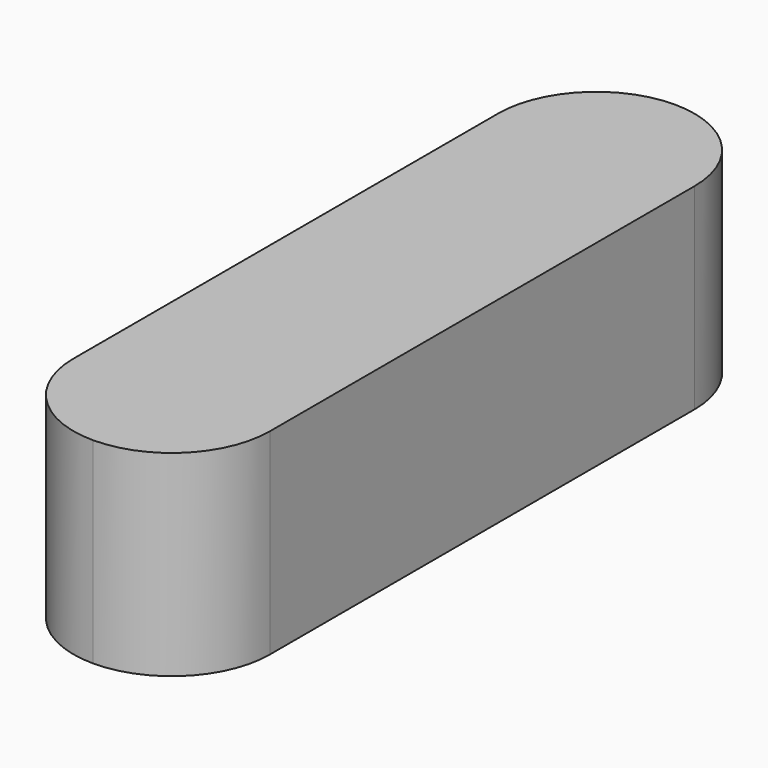
from build123d import *

# Parameters (mm, degrees)
F0_W     = 10
F0_H     = 37
F1_DEPTH = 10
F2_R     = 4.99999


# Not quite as in the source:
# - a fillet or chamfer is up to 0.001 mm smaller than in the source, because OpenCascade refuses the exact size


with BuildPart() as f1:
    # F0 (on Top) → F1 (new body)
    with BuildSketch(Plane.XY):
        Rectangle(F0_W, F0_H)
    extrude(amount=F1_DEPTH)

    # F2 (radius 5 in the source; OpenCascade refuses exactly that, so slightly less here)
    f2_edges = [f1.edges().sort_by_distance(p)[0] for p in [
        (-5, 18.5, 5),
        (5, 18.5, 5),
        (-5, -18.5, 5),
        (5, -18.5, 5),
    ]]
    fillet(f2_edges, radius=F2_R)


solid = f1.part
